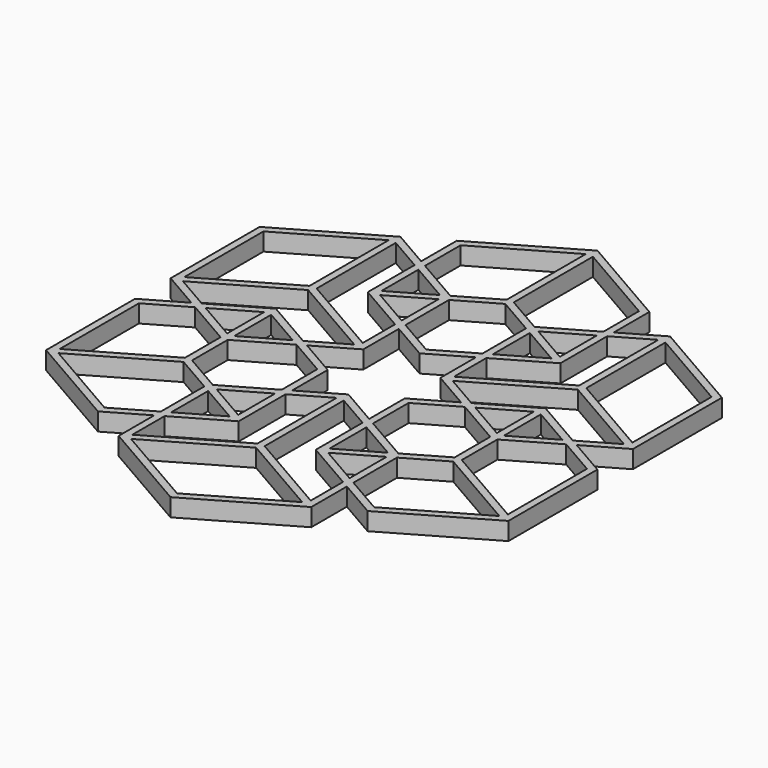
from build123d import *

# Parameters (mm, degrees)
F1_DEPTH = 2


# Not quite as in the source:
# - a feature names something its author has since deleted; it is built from what else it names


with BuildPart() as f1:
    # F0 (on Top) → F1 (new body)
    with BuildSketch(Plane.XY):
        Polygon((-15.1554445662, 3.75), (-20.8506350946, 0.4618802154), (-20.0506350946, 0), (-15.5554445662, 2.5952994616), (-15.5554445662, -2.5952994616), (-15.1554445662, -2.8262395693), (-14.7554445662, -2.5952994616), (-14.7554445662, 2.5952994616), (-10.2602540378, 0), (-9.4602540378, 0.4618802154), align=None)
        Polygon((-15.1554445662, -21.25), (-10.8253175473, -18.75), (-10.8253175473, -17.8262395693), (-15.1554445662, -20.3262395693), (-24.7807621135, -14.7690598923), (-15.1554445662, -9.2118802154), (-10.8253175473, -11.7118802154), (-10.8253175473, -11.25), (-10.4253175473, -11.0190598923), (-14.7554445662, -8.5190598923), (-14.7554445662, -3.5190598923), (-15.1554445662, -3.75), (-15.5554445662, -3.5190598923), (-15.5554445662, -8.5190598923), (-25.1807621135, -14.0762395693), (-25.1807621135, -2.9618802154), (-20.8506350946, -0.4618802154), (-21.6506350946, 0), (-25.9807621135, -2.5), (-25.9807621135, -15), align=None)
        Polygon((-10.0253175473, -17.3643593539), (-10.0253175473, -18.2881197846), (-4.3301270189, -15), (-4.3301270189, -8.4237604307), (-5.1301270189, -8.8856406461), (-5.1301270189, -14.0762395693), (-9.6253175473, -11.4809401077), (-10.0253175473, -11.7118802154), (-10.0253175473, -12.1737604307), (-5.5301270189, -14.7690598923), align=None)
        Polygon((-5.1301270189, -7.9618802154), (-4.3301270189, -7.5), (-4.3301270189, -2.5), (-8.6602540378, 0), (-9.4602540378, -0.4618802154), (-5.1301270189, -2.9618802154), align=None)
        Polygon((-14.7554445662, -2.5952994616), (-14.7554445662, -3.5190598923), (-9.4602540378, -0.4618802154), (-10.2602540378, 0), align=None)
        Polygon((-20.0506350946, 0), (-20.8506350946, -0.4618802154), (-15.5554445662, -3.5190598923), (-15.5554445662, -2.5952994616), align=None)
        Polygon((-15.1554445662, -3.75), (-14.7554445662, -3.5190598923), (-14.7554445662, -2.5952994616), (-15.1554445662, -2.8262395693), (-15.5554445662, -2.5952994616), (-15.5554445662, -3.5190598923), align=None)
        Polygon((-20.8506350946, 0.4618802154), (-21.6506350946, 0), (-20.8506350946, -0.4618802154), (-20.0506350946, 0), align=None)
        Polygon((-9.4602540378, -0.4618802154), (-8.6602540378, 0), (-9.4602540378, 0.4618802154), (-10.2602540378, 0), align=None)
        Polygon((-25.9807621135, 2.5), (-21.6506350946, 0), (-20.8506350946, 0.4618802154), (-24.7807621135, 2.7309401077), (-15.1554445662, 8.2881197846), (-5.5301270189, 2.7309401077), (-9.4602540378, 0.4618802154), (-8.6602540378, 0), (-4.3301270189, 2.5), (-4.3301270189, 7.5), (-5.1301270189, 7.9618802154), (-5.1301270189, 3.4237604307), (-14.7554445662, 8.9809401077), (-14.7554445662, 20.0952994616), (-10.8253175473, 17.8262395693), (-10.8253175473, 18.75), (-15.1554445662, 21.25), (-25.9807621135, 15), align=None)
        Polygon((-15.5554445662, 8.9809401077), (-25.1807621135, 3.4237604307), (-25.1807621135, 14.5381197846), (-15.5554445662, 20.0952994616), align=None, mode=Mode.SUBTRACT)
        Polygon((-5.1301270189, -7.9618802154), (-10.4253175473, -11.0190598923), (-9.6253175473, -11.4809401077), (-5.1301270189, -8.8856406461), align=None)
        Polygon((-5.1301270189, -8.8856406461), (-4.3301270189, -8.4237604307), (-4.3301270189, -7.5), (-5.1301270189, -7.9618802154), align=None)
        Polygon((-10.8253175473, -11.7118802154), (-10.8253175473, -17.8262395693), (-10.0253175473, -17.3643593539), (-10.0253175473, -12.1737604307), align=None)
        Polygon((-10.8253175473, -11.25), (-10.8253175473, -11.7118802154), (-10.0253175473, -12.1737604307), (-10.0253175473, -11.7118802154), (-9.6253175473, -11.4809401077), (-10.4253175473, -11.0190598923), align=None)
        Polygon((-10.8253175473, -23.75), (0, -30), (10.8253175473, -23.75), (10.8253175473, -18.75), (10.0253175473, -18.2881197846), (10.0253175473, -22.8262395693), (0.4, -17.2690598923), (0.4, -6.1547005384), (4.3301270189, -8.4237604307), (4.3301270189, -7.5), (0, -5), (-4.3301270189, -7.5), (-4.3301270189, -8.4237604307), (-0.4, -6.1547005384), (-0.4, -17.2690598923), (-10.0253175473, -22.8262395693), (-10.0253175473, -18.2881197846), (-10.8253175473, -18.75), align=None)
        Polygon((0, -17.9618802154), (9.6253175473, -23.5190598923), (0, -29.0762395693), (-9.6253175473, -23.5190598923), align=None, mode=Mode.SUBTRACT)
        Polygon((-10.8253175473, -17.8262395693), (-10.8253175473, -18.75), (-10.0253175473, -18.2881197846), (-10.0253175473, -17.3643593539), align=None)
        Polygon((-10.8253175473, 11.25), (-5.1301270189, 7.9618802154), (-5.1301270189, 8.8856406461), (-9.6253175473, 11.4809401077), (-5.1301270189, 14.0762395693), (-5.1301270189, 14.5381197846), (-5.5301270189, 14.7690598923), (-10.0253175473, 12.1737604307), (-10.0253175473, 17.3643593539), (-10.8253175473, 17.8262395693), align=None)
        Polygon((-5.1301270189, 7.9618802154), (-4.3301270189, 7.5), (-4.3301270189, 8.4237604307), (-5.1301270189, 8.8856406461), align=None)
        Polygon((-5.1301270189, 8.8856406461), (-4.3301270189, 8.4237604307), (-4.3301270189, 14.5381197846), (-5.1301270189, 14.0762395693), align=None)
        Polygon((-4.7301270189, 15.2309401077), (-10.0253175473, 18.2881197846), (-10.0253175473, 17.3643593539), (-5.5301270189, 14.7690598923), align=None)
        Polygon((-10.0253175473, 18.2881197846), (-10.8253175473, 18.75), (-10.8253175473, 17.8262395693), (-10.0253175473, 17.3643593539), align=None)
        Polygon((-5.1301270189, 14.0762395693), (-4.3301270189, 14.5381197846), (-4.3301270189, 15), (-4.7301270189, 15.2309401077), (-5.5301270189, 14.7690598923), (-5.1301270189, 14.5381197846), align=None)
        Polygon((-10.8253175473, 23.75), (-10.8253175473, 18.75), (-10.0253175473, 18.2881197846), (-10.0253175473, 23.2881197846), (-0.4, 28.8452994616), (-0.4, 17.7309401077), (-4.7301270189, 15.2309401077), (-4.3301270189, 15), (-4.3301270189, 14.5381197846), (0, 17.0381197846), (4.3301270189, 14.5381197846), (4.3301270189, 15), (4.7301270189, 15.2309401077), (0.4, 17.7309401077), (0.4, 28.8452994616), (10.0253175473, 23.2881197846), (10.0253175473, 18.2881197846), (10.8253175473, 18.75), (10.8253175473, 23.75), (0, 30), align=None)
        Polygon((-4.3301270189, 8.4237604307), (-4.3301270189, 7.5), (0, 5), (4.3301270189, 7.5), (4.3301270189, 8.4237604307), (0, 5.9237604307), align=None)
        Polygon((4.3301270189, 8.4237604307), (4.3301270189, 7.5), (5.1301270189, 7.9618802154), (5.1301270189, 8.8856406461), align=None)
        Polygon((4.3301270189, 14.5381197846), (4.3301270189, 8.4237604307), (5.1301270189, 8.8856406461), (5.1301270189, 14.0762395693), align=None)
        Polygon((10.8253175473, 11.25), (10.8253175473, 17.8262395693), (10.0253175473, 17.3643593539), (10.0253175473, 12.1737604307), (5.5301270189, 14.7690598923), (5.1301270189, 14.5381197846), (5.1301270189, 14.0762395693), (9.6253175473, 11.4809401077), (5.1301270189, 8.8856406461), (5.1301270189, 7.9618802154), align=None)
        Polygon((5.5301270189, 14.7690598923), (4.7301270189, 15.2309401077), (4.3301270189, 15), (4.3301270189, 14.5381197846), (5.1301270189, 14.0762395693), (5.1301270189, 14.5381197846), align=None)
        Polygon((10.0253175473, 17.3643593539), (10.0253175473, 18.2881197846), (4.7301270189, 15.2309401077), (5.5301270189, 14.7690598923), align=None)
        Polygon((20.8506350946, 0.4618802154), (21.6506350946, 0), (25.9807621135, 2.5), (25.9807621135, 15), (15.1554445662, 21.25), (10.8253175473, 18.75), (10.8253175473, 17.8262395693), (14.7554445662, 20.0952994616), (14.7554445662, 8.9809401077), (5.1301270189, 3.4237604307), (5.1301270189, 7.9618802154), (4.3301270189, 7.5), (4.3301270189, 2.5), (8.6602540378, 0), (9.4602540378, 0.4618802154), (5.5301270189, 2.7309401077), (15.1554445662, 8.2881197846), (24.7807621135, 2.7309401077), align=None)
        Polygon((15.5554445662, 8.9809401077), (15.5554445662, 20.0952994616), (25.1807621135, 14.5381197846), (25.1807621135, 3.4237604307), align=None, mode=Mode.SUBTRACT)
        Polygon((10.8253175473, 17.8262395693), (10.8253175473, 18.75), (10.0253175473, 18.2881197846), (10.0253175473, 17.3643593539), align=None)
        Polygon((9.4602540378, -0.4618802154), (14.7554445662, -3.5190598923), (14.7554445662, -2.5952994616), (10.2602540378, 0), align=None)
        Polygon((9.4602540378, 0.4618802154), (8.6602540378, 0), (9.4602540378, -0.4618802154), (10.2602540378, 0), align=None)
        Polygon((20.0506350946, 0), (20.8506350946, 0.4618802154), (15.1554445662, 3.75), (9.4602540378, 0.4618802154), (10.2602540378, 0), (14.7554445662, 2.5952994616), (14.7554445662, -2.5952994616), (15.1554445662, -2.8262395693), (15.5554445662, -2.5952994616), (15.5554445662, 2.5952994616), align=None)
        Polygon((14.7554445662, -2.5952994616), (14.7554445662, -3.5190598923), (15.1554445662, -3.75), (15.5554445662, -3.5190598923), (15.5554445662, -2.5952994616), (15.1554445662, -2.8262395693), align=None)
        Polygon((15.5554445662, -3.5190598923), (20.8506350946, -0.4618802154), (20.0506350946, 0), (15.5554445662, -2.5952994616), align=None)
        Polygon((20.8506350946, -0.4618802154), (21.6506350946, 0), (20.8506350946, 0.4618802154), (20.0506350946, 0), align=None)
        Polygon((10.8253175473, -17.8262395693), (10.8253175473, -18.75), (15.1554445662, -21.25), (25.9807621135, -15), (25.9807621135, -2.5), (21.6506350946, 0), (20.8506350946, -0.4618802154), (25.1807621135, -2.9618802154), (25.1807621135, -14.0762395693), (15.5554445662, -8.5190598923), (15.5554445662, -3.5190598923), (15.1554445662, -3.75), (14.7554445662, -3.5190598923), (14.7554445662, -8.5190598923), (10.4253175473, -11.0190598923), (10.8253175473, -11.25), (10.8253175473, -11.7118802154), (15.1554445662, -9.2118802154), (24.7807621135, -14.7690598923), (15.1554445662, -20.3262395693), align=None)
        Polygon((4.3301270189, -2.5), (4.3301270189, -7.5), (5.1301270189, -7.9618802154), (5.1301270189, -2.9618802154), (9.4602540378, -0.4618802154), (8.6602540378, 0), align=None)
        Polygon((4.3301270189, -7.5), (4.3301270189, -8.4237604307), (5.1301270189, -8.8856406461), (5.1301270189, -7.9618802154), align=None)
        Polygon((9.6253175473, -11.4809401077), (10.4253175473, -11.0190598923), (5.1301270189, -7.9618802154), (5.1301270189, -8.8856406461), align=None)
        Polygon((4.3301270189, -15), (10.0253175473, -18.2881197846), (10.0253175473, -17.3643593539), (5.5301270189, -14.7690598923), (10.0253175473, -12.1737604307), (10.0253175473, -11.7118802154), (9.6253175473, -11.4809401077), (5.1301270189, -14.0762395693), (5.1301270189, -8.8856406461), (4.3301270189, -8.4237604307), align=None)
        Polygon((10.0253175473, -17.3643593539), (10.8253175473, -17.8262395693), (10.8253175473, -11.7118802154), (10.0253175473, -12.1737604307), align=None)
        Polygon((10.0253175473, -18.2881197846), (10.8253175473, -18.75), (10.8253175473, -17.8262395693), (10.0253175473, -17.3643593539), align=None)
        Polygon((10.0253175473, -12.1737604307), (10.8253175473, -11.7118802154), (10.8253175473, -11.25), (10.4253175473, -11.0190598923), (9.6253175473, -11.4809401077), (10.0253175473, -11.7118802154), align=None)
    extrude(amount=F1_DEPTH)


solid = f1.part
